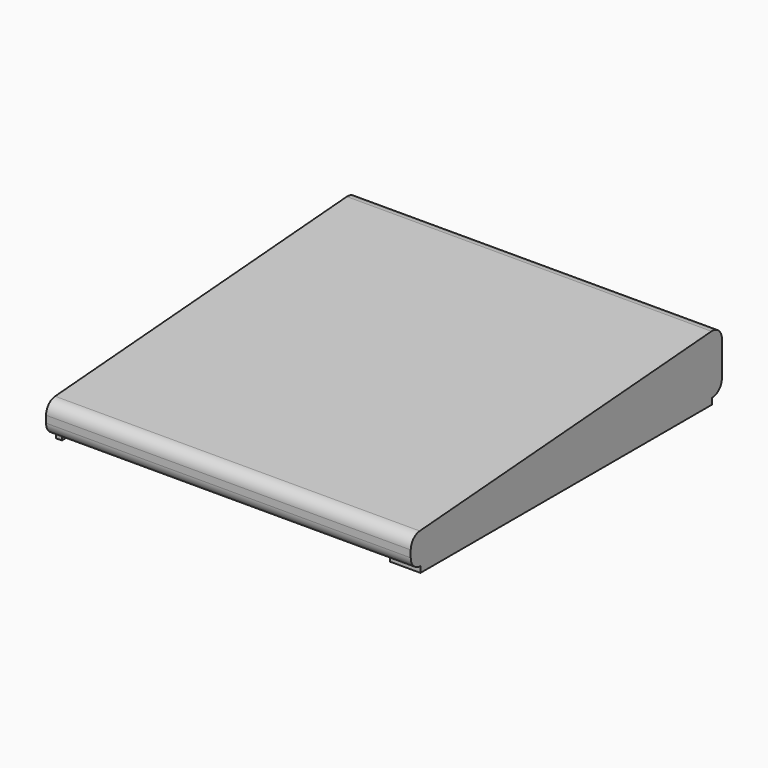
from build123d import *

# Parameters (mm, degrees)
F1_DEPTH = 300
F2_T     = -5
F4_DEPTH = 25
F7_DEPTH = 5
F9_DEPTH = 300


# Not quite as in the source:
# - a feature of the source that left no trace in its solid (it failed there, or was rolled back) is left out
# - a feature names something its author has since deleted; it is built from what else it names


with BuildPart() as f1:
    # F0 (on Right) → F1 (new body)
    with BuildSketch(Plane.YZ):
        with BuildLine():
            ThreePointArc((-361.3383226016, -15), (-358.4093904135, -22.0710678119), (-351.3383226016, -25))
            Line((-351.3383226016, -25), (-51.3383226016, -25))
            ThreePointArc((-51.3383226016, -25), (-44.2672547897, -22.0710678119), (-41.3383226016, -15))
            Line((-41.3383226016, -15), (-41.3383226016, 13.3530771738))
            ThreePointArc((-41.3383226016, 13.3530771738), (-44.538361228, 20.6852341086), (-52.0904276652, 23.3247539622))
            Line((-52.0904276652, 23.3247539622), (-352.0904276652, 0.6975144458))
            ThreePointArc((-352.0904276652, 0.6975144458), (-358.6704795365, -2.474200969), (-361.3383226016, -9.2741623426))
            Line((-361.3383226016, -9.2741623426), (-361.3383226016, -15))
        make_face()
    extrude(amount=F1_DEPTH)

    # F2: a shell. OpenCascade refuses it in one call, so the cavity is built on its own and cut out:
    # the body offset inwards by the wall thickness, plus a prism from it out through each open face.
    f2_core = offset(f1.part, amount=F2_T, mode=Mode.PRIVATE)
    f2_exits = [f2_core.faces().sort_by_distance(p)[0] for p in [
        (150, -201.338323, -20),
    ]]
    add(f2_core, mode=Mode.SUBTRACT)
    extrude(f2_exits, amount=-F2_T, mode=Mode.SUBTRACT)

    # F4 (add): a face of the model
    f4_faces = [f1.faces().sort_by_distance(p)[0] for p in [
        (300, -183.9481701293, -5.8146709921),
    ]]
    extrude(f4_faces, amount=-F4_DEPTH)

    # F7 (add): faces of the model
    f7_faces = [f1.faces().sort_by_distance(p)[0] for p in [
        (2.5, -201.3383226016, -25),
        (287.5, -201.3383226016, -25),
    ]]
    extrude(f7_faces, amount=F7_DEPTH)

    # F0 (on Right) → F9 (cut)
    with BuildSketch(Plane.YZ):
        with BuildLine():
            ThreePointArc((-361.3383226016, -15), (-358.4093904135, -22.0710678119), (-351.3383226016, -25))
            Line((-351.3383226016, -25), (-51.3383226016, -25))
            ThreePointArc((-51.3383226016, -25), (-44.2672547897, -22.0710678119), (-41.3383226016, -15))
            Line((-41.3383226016, -15), (-41.3383226016, 13.3530771738))
            ThreePointArc((-41.3383226016, 13.3530771738), (-44.538361228, 20.6852341086), (-52.0904276652, 23.3247539622))
            Line((-52.0904276652, 23.3247539622), (-352.0904276652, 0.6975144458))
            ThreePointArc((-352.0904276652, 0.6975144458), (-358.6704795365, -2.474200969), (-361.3383226016, -9.2741623426))
            Line((-361.3383226016, -9.2741623426), (-361.3383226016, -15))
        make_face()
    extrude(amount=-F9_DEPTH, mode=Mode.SUBTRACT)


solid = f1.part
